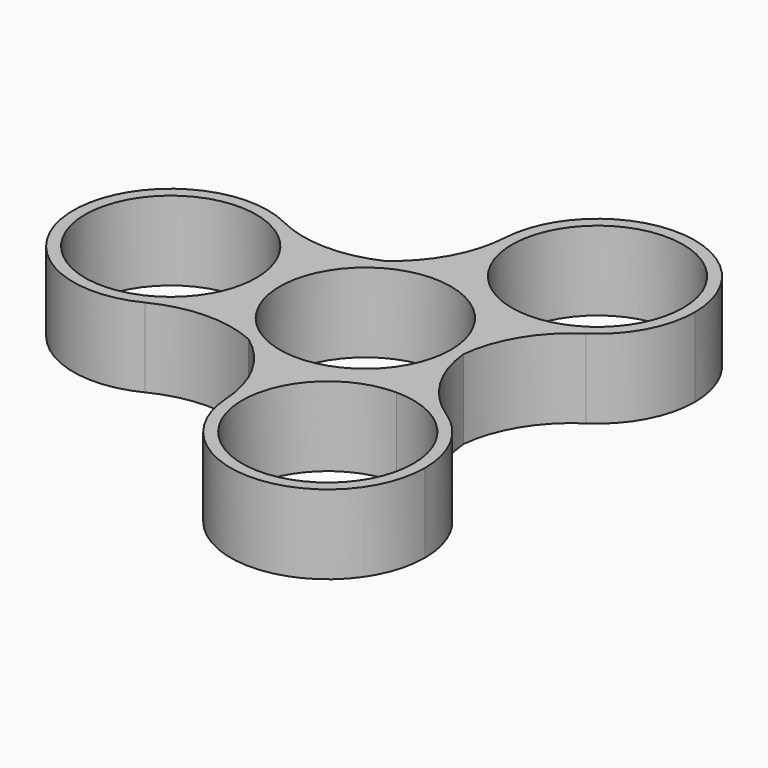
from build123d import *

# Parameters (mm, degrees)
F0_R        = 11
F1_DEPTH    = 10.16
F2_T1_DEPTH = 10.16


# Not quite as in the source:
# - a fillet or chamfer that OpenCascade refuses, or shapes differently, is made with other operations: its cross-section is extruded or revolved along the edge and cut away or added


with BuildPart() as f1:
    # F0 (on Top) → F1 (new body)
    with BuildSketch(Plane.XY):
        with BuildLine():
            ThreePointArc((-6.2500001721, -10.8253174479), (-12.5, 3.1e-08), (-6.2500001185, 10.8253174789))
            Line((-6.2500001185, 10.8253174789), (-14.177453734, 6.2484))
            ThreePointArc((-14.177453734, 6.2484), (-12.929018134, 3.2344098428), (-12.5032, 0))
            ThreePointArc((-12.5032, 0), (-12.929018134, -3.2344098428), (-14.177453734, -6.2484))
            Line((-14.177453734, -6.2484), (-6.2500001721, -10.8253174479))
        make_face()
        with BuildLine():
            Line((-15.4737205584, 5.5), (-14.177453734, 6.2484))
            ThreePointArc((-14.177453734, 6.2484), (-37.4968, 0), (-14.177453734, -6.2484))
            Line((-14.177453734, -6.2484), (-15.4737205584, -5.5))
            ThreePointArc((-15.4737205584, -5.5), (-36, 0), (-15.4737205584, 5.5))
        make_face()
        with BuildLine():
            Line((12.5, -9.1538350946), (12.5, 0))
            ThreePointArc((12.5, 0), (6.2499999139, -10.825317597), (-6.2500001721, -10.8253174479))
            Line((-6.2500001721, -10.8253174479), (1.677453734, -15.4022350946))
            ThreePointArc((1.677453734, -15.4022350946), (6.2516, -10.8280888286), (12.5, -9.1538350946))
        make_face()
        with BuildLine():
            ThreePointArc((24.9968, -21.6506350946), (21.3365720231, -12.8140630715), (12.5, -9.1538350946))
            Line((12.5, -9.1538350946), (12.5, -10.6506350946))
            ThreePointArc((12.5, -10.6506350946), (20.2781745931, -13.8724605016), (23.5, -21.6506350946))
            ThreePointArc((23.5, -21.6506350946), (9.6529905039, -32.2758191838), (2.9737205584, -16.1506350946))
            Line((2.9737205584, -16.1506350946), (1.677453734, -15.4022350946))
            ThreePointArc((1.677453734, -15.4022350946), (9.2655901572, -33.7216169606), (24.9968, -21.6506350946))
        make_face()
        with BuildLine():
            Line((12.5, -10.6506350946), (12.5, -9.1538350946))
            ThreePointArc((12.5, -9.1538350946), (6.2516, -10.8280888286), (1.677453734, -15.4022350946))
            Line((1.677453734, -15.4022350946), (2.9737205584, -16.1506350946))
            ThreePointArc((2.9737205584, -16.1506350946), (7, -12.124355653), (12.5, -10.6506350946))
        make_face()
        with BuildLine():
            ThreePointArc((-6.2500001721, -10.8253174479), (6.2499999139, -10.825317597), (12.5, 0))
            ThreePointArc((12.5, 0), (6.2499999408, 10.8253175815), (-6.2500001185, 10.8253174789))
            ThreePointArc((-6.2500001185, 10.8253174789), (-12.5, 3.1e-08), (-6.2500001721, -10.8253174479))
        make_face()
        Circle(F0_R, mode=Mode.SUBTRACT)
        with BuildLine():
            ThreePointArc((-6.2500001185, 10.8253174789), (6.2499999408, 10.8253175815), (12.5, 0))
            Line((12.5, 0), (12.5, 9.1538350946))
            ThreePointArc((12.5, 9.1538350946), (6.2516, 10.8280888286), (1.677453734, 15.4022350946))
            Line((1.677453734, 15.4022350946), (-6.2500001185, 10.8253174789))
        make_face()
        with BuildLine():
            ThreePointArc((1.677453734, 15.4022350946), (6.2516, 10.8280888286), (12.5, 9.1538350946))
            Line((12.5, 9.1538350946), (12.5, 10.6506350946))
            ThreePointArc((12.5, 10.6506350946), (7, 12.124355653), (2.9737205584, 16.1506350946))
            Line((2.9737205584, 16.1506350946), (1.677453734, 15.4022350946))
        make_face()
        with BuildLine():
            Line((12.5, 10.6506350946), (12.5, 9.1538350946))
            ThreePointArc((12.5, 9.1538350946), (21.3365720231, 12.8140630715), (24.9968, 21.6506350946))
            ThreePointArc((24.9968, 21.6506350946), (9.2655901572, 33.7216169606), (1.677453734, 15.4022350946))
            Line((1.677453734, 15.4022350946), (2.9737205584, 16.1506350946))
            ThreePointArc((2.9737205584, 16.1506350946), (9.6529905039, 32.2758191838), (23.5, 21.6506350946))
            ThreePointArc((23.5, 21.6506350946), (20.2781745931, 13.8724605016), (12.5, 10.6506350946))
        make_face()
        with BuildLine():
            ThreePointArc((-12.5032, 0), (-12.929018134, 3.2344098428), (-14.177453734, 6.2484))
            Line((-14.177453734, 6.2484), (-15.4737205584, 5.5))
            ThreePointArc((-15.4737205584, 5.5), (-14.3748159108, 2.8470094961), (-14, 0))
            ThreePointArc((-14, 0), (-14.3748159108, -2.8470094961), (-15.4737205584, -5.5))
            Line((-15.4737205584, -5.5), (-14.177453734, -6.2484))
            ThreePointArc((-14.177453734, -6.2484), (-12.929018134, -3.2344098428), (-12.5032, 0))
        make_face()
    extrude(amount=F1_DEPTH)

    # F2: fillet of radius 15.24 on 6 edges, made by hand

    # F2_s2 → F2_t1 (join)
    with BuildSketch(Plane.XY):
        with BuildLine():
            ThreePointArc((-4.9300135605, -11.5874120735), (-12.1072951031, -9.5520710185), (-19.3906654504, -11.1671561353))
            ThreePointArc((-19.3906654504, -11.1671561353), (-16.42385767, -9.0895430565), (-14.177453734, -6.2484))
            Line((-14.177453734, -6.2484), (-4.9300135605, -11.5874120735))
        make_face()
        with BuildLine():
            ThreePointArc((12.5, -1.5241890523), (14.3259837123, 5.7091896211), (19.3663736264, 11.2092308086))
            ThreePointArc((19.3663736264, 11.2092308086), (16.0837040307, 9.6787064421), (12.5, 9.1538350946))
            Line((12.5, 9.1538350946), (12.5, -1.5241890523))
        make_face()
        with BuildLine():
            ThreePointArc((19.3663736264, -11.2092308086), (14.3259837123, -5.7091896211), (12.5, 1.5241890523))
            Line((12.5, 1.5241890523), (12.5, -9.1538350946))
            ThreePointArc((12.5, -9.1538350946), (16.0837040307, -9.6787064421), (19.3663736264, -11.2092308086))
        make_face()
        with BuildLine():
            ThreePointArc((0.024291824, 22.3763869439), (-2.2186886092, 15.2612606396), (-7.5699864395, 10.0632230212))
            Line((-7.5699864395, 10.0632230212), (1.677453734, 15.4022350946))
            ThreePointArc((1.677453734, 15.4022350946), (0.3401536393, 18.7682494986), (0.024291824, 22.3763869439))
        make_face()
        with BuildLine():
            ThreePointArc((-4.9300135605, 11.5874120735), (-12.1072951031, 9.5520710185), (-19.3906654504, 11.1671561353))
            ThreePointArc((-19.3906654504, 11.1671561353), (-16.42385767, 9.0895430565), (-14.177453734, 6.2484))
            Line((-14.177453734, 6.2484), (-4.9300135605, 11.5874120735))
        make_face()
        with BuildLine():
            ThreePointArc((-7.5699864395, -10.0632230212), (-2.2186886092, -15.2612606396), (0.024291824, -22.3763869439))
            ThreePointArc((0.024291824, -22.3763869439), (0.3401536393, -18.7682494986), (1.677453734, -15.4022350946))
            Line((1.677453734, -15.4022350946), (-7.5699864395, -10.0632230212))
        make_face()
    extrude(amount=F2_T1_DEPTH)


solid = f1.part
